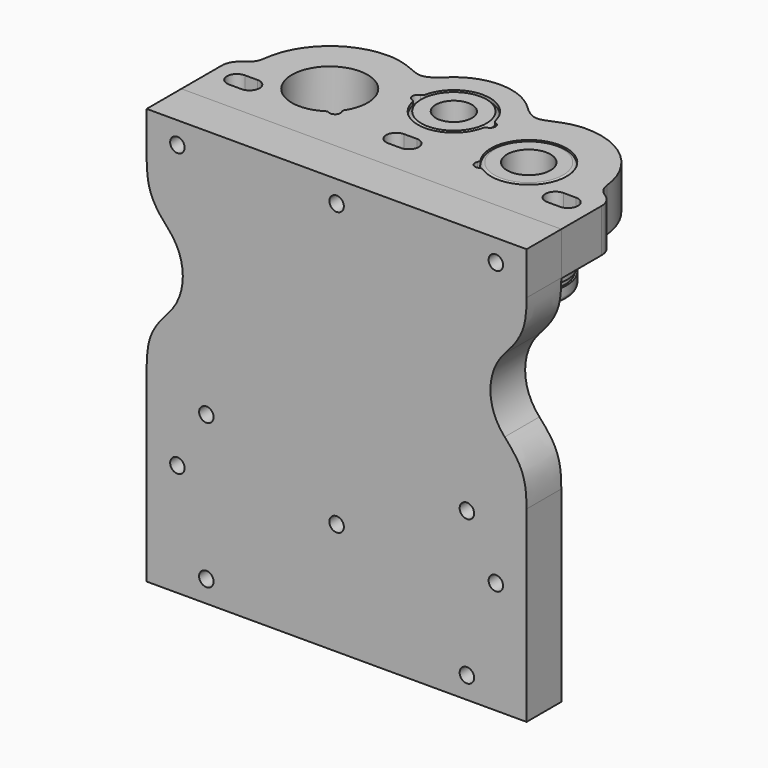
from build123d import *

# Parameters (mm, degrees)
F0_W         = 105
F0_H         = 90
F1_DEPTH     = 12
F3_DEPTH     = 12
F4_R         = 5
F5_R         = 10.5
F5_R_2       = 6
F6_DEPTH     = 30
F8_START     = -3.5
F7_R         = 13.9480454754
F7_R_2       = 10
F8_DEPTH     = 1.3
F10_START    = -3.5
F9_R         = 14.6955703702
F9_R_2       = 10
F10_DEPTH    = 1.3
F11_R        = 1
F12_W        = 105
F12_H        = 25
F13_DEPTH    = 12
F14_R        = 10
F14_R_2      = 5
F15_DEPTH    = 25
F16_R        = 2
F17_DEPTH    = 25
F18_SIZE     = 1
F19_R        = 15
F20_DEPTH    = 25
F21_T1_DEPTH = 69.741647668


# Not quite as in the source:
# - a fillet or chamfer that OpenCascade refuses, or shapes differently, is made with other operations: its cross-section is extruded or revolved along the edge and cut away or added


with BuildPart() as f1:
    # F0 (on Front) → F1 (new body)
    with BuildSketch(Plane.XZ):
        with Locations((0, 45)):
            Rectangle(F0_W, F0_H)
    extrude(amount=-F1_DEPTH)

    # F12 (on face) → F13 (join, through all)
    with BuildSketch(Plane.XZ):
        with Locations((0, -12.5)):
            Rectangle(F12_W, F12_H)
    extrude(amount=-F13_DEPTH)


with BuildPart() as f3:
    # F2 (on face) → F3 (new body)
    with BuildSketch(Plane.XY.offset(90)):
        with BuildLine():
            Line((52.5, 28.5), (47.4999980907, 32))
            ThreePointArc((47.4999980907, 32), (41.6421337144, 46.1421356237), (27.4999980907, 52))
            add(Edge.make_bspline(
                [(11.1242977306, 52), (13.1569224157, 50.0337806808), (16.8978786945, 47.5177026437), (21.9085912172, 52), (27.4999980907, 52)],
                knots=[0, 0, 0, 0, 0.4241441638, 1, 1, 1, 1], degree=3))
            ThreePointArc((11.1242977306, 52), (0, 56.5), (-11.1242977306, 52))
            add(Edge.make_bspline(
                [(-11.1242977306, 52), (-13.1569224157, 50.0337806808), (-16.8978786945, 47.5177026437), (-21.9085912172, 52), (-27.4999980907, 52)],
                knots=[0, 0, 0, 0, 0.4241441638, 1, 1, 1, 1], degree=3))
            ThreePointArc((-27.4999980907, 52), (-41.6421337144, 46.1421356237), (-47.4999980907, 32))
            Line((-47.4999980907, 32), (-52.5, 28.5))
            Line((-52.5, 28.5), (-52.5, 12))
            Line((-52.5, 12), (-47.5, 12))
            Line((-47.5, 12), (47.5, 12))
            Line((47.5, 12), (52.5, 12))
            Line((52.5, 12), (52.5, 28.5))
        make_face()
        with BuildLine():
            Line((-45.75, 25.5), (-42.25, 25.5))
            ThreePointArc((-42.25, 25.5), (-39.5, 22.75), (-42.25, 20))
            Line((-42.25, 20), (-45.75, 20))
            ThreePointArc((-45.75, 20), (-48.5, 22.75), (-45.75, 25.5))
        make_face(mode=Mode.SUBTRACT)
        with BuildLine():
            ThreePointArc((-20.7869945386, 23.2632266648), (-21.2971382344, 23.3755438907), (-21.794316347, 23.2153075842))
            ThreePointArc((-21.794316347, 23.2153075842), (-34.9069416236, 39.4069435329), (-18.7153056748, 26.2943182564))
            ThreePointArc((-18.7153056748, 26.2943182564), (-18.8755419814, 25.7971401438), (-18.7632247555, 25.286996448))
            ThreePointArc((-18.7632247555, 25.286996448), (-19.0323943859, 23.5323962953), (-20.7869945386, 23.2632266648))
        make_face(mode=Mode.SUBTRACT)
        with BuildLine():
            ThreePointArc((-1.75, 20), (-4.5, 22.75), (-1.75, 25.5))
            Line((-1.75, 25.5), (1.75, 25.5))
            ThreePointArc((1.75, 25.5), (4.5, 22.75), (1.75, 20))
            Line((1.75, 20), (-1.75, 20))
        make_face(mode=Mode.SUBTRACT)
        with BuildLine():
            ThreePointArc((42.25, 20), (39.5, 22.75), (42.25, 25.5))
            Line((42.25, 25.5), (45.75, 25.5))
            ThreePointArc((45.75, 25.5), (48.5, 22.75), (45.75, 20))
            Line((45.75, 20), (42.25, 20))
        make_face(mode=Mode.SUBTRACT)
        with BuildLine():
            ThreePointArc((18.7153056748, 26.2943182564), (34.9069416236, 39.4069435329), (21.794316347, 23.2153075842))
            ThreePointArc((21.794316347, 23.2153075842), (21.2971382344, 23.3755438907), (20.7869945386, 23.2632266648))
            ThreePointArc((20.7869945386, 23.2632266648), (19.0323943859, 23.5323962953), (18.7632247555, 25.286996448))
            ThreePointArc((18.7632247555, 25.286996448), (18.8755419814, 25.7971401438), (18.7153056748, 26.2943182564))
        make_face(mode=Mode.SUBTRACT)
        with BuildLine():
            ThreePointArc((9.7358200456, 38.3287254802), (0, 30.525), (-9.7358200456, 38.3287254802))
            ThreePointArc((-9.7358200456, 38.3287254802), (-9.9771083652, 38.7894094573), (-10.4171052632, 39.0666323095))
            ThreePointArc((-10.4171052632, 39.0666323095), (-11.475, 40.5), (-10.4171052632, 41.9333676905))
            ThreePointArc((-10.4171052632, 41.9333676905), (-9.9771083652, 42.2105905427), (-9.7358200456, 42.6712745198))
            ThreePointArc((-9.7358200456, 42.6712745198), (0, 50.475), (9.7358200456, 42.6712745198))
            ThreePointArc((9.7358200456, 42.6712745198), (9.9771083652, 42.2105905427), (10.4171052632, 41.9333676905))
            ThreePointArc((10.4171052632, 41.9333676905), (11.475, 40.5), (10.4171052632, 39.0666323095))
            ThreePointArc((10.4171052632, 39.0666323095), (9.9771083652, 38.7894094573), (9.7358200456, 38.3287254802))
        make_face(mode=Mode.SUBTRACT)
    extrude(amount=-F3_DEPTH)

    # F4
    f4_edges = [f3.edges().sort_by_distance(p)[0] for p in [
        (-47.499998, 32, 84),
        (-52.5, 28.5, 84),
        (47.499998, 32, 84),
        (52.5, 28.5, 84),
    ]]
    fillet(f4_edges, radius=F4_R)


with BuildPart() as f6:
    # F5 (on face) → F6 (new body)
    with BuildSketch(Plane.XY.offset(90)):
        with Locations((27.4999980907, 32)):
            Circle(F5_R)
        with Locations((27.4999980907, 32)):
            Circle(F5_R_2, mode=Mode.SUBTRACT)
    extrude(amount=-F6_DEPTH)

    # F7 (on face) → F8 (cut)
    with BuildSketch(Plane.XY.offset(90).offset(F8_START)):
        with Locations((27.4999980907, 32)):
            Circle(F7_R)
        with Locations((27.4999980907, 32)):
            Circle(F7_R_2, mode=Mode.SUBTRACT)
    extrude(amount=-F8_DEPTH, mode=Mode.SUBTRACT)

    # F9 (on face) → F10 (cut)
    with BuildSketch(Plane(origin=(0, 0, 60), x_dir=(1, 0, 0), z_dir=(0, 0, -1)).offset(F10_START)):
        with Locations((27.4999980907, -32)):
            Circle(F9_R)
        with Locations((27.4999980907, -32)):
            Circle(F9_R_2, mode=Mode.SUBTRACT)
    extrude(amount=-F10_DEPTH, mode=Mode.SUBTRACT)

    # F11
    f11_edges = [f6.edges().sort_by_distance(p)[0] for p in [
        (16.999998, 32, 90),
        (16.999998, 32, 60),
    ]]
    fillet(f11_edges, radius=F11_R)


with BuildPart() as f15:
    # F14 (on face) → F15 (new body)
    with BuildSketch(Plane.XY.offset(90)):
        with Locations((0, 40.5)):
            Circle(F14_R)
        with Locations((0, 40.5)):
            Circle(F14_R_2, mode=Mode.SUBTRACT)
    extrude(amount=-F15_DEPTH)

    # F18
    f18_edges = [f15.edges().sort_by_distance(p)[0] for p in [
        (-10, 40.5, 65),
        (-10, 40.5, 90),
    ]]
    chamfer(f18_edges, length=F18_SIZE)


with BuildPart() as f17_tool:
    # F16 (on face) → F17 (new body)
    with BuildSketch(Plane.XZ):
        with Locations((-44, 84)):
            Circle(F16_R)
        with Locations((44, 84)):
            Circle(F16_R)
        with Locations((0, 84)):
            Circle(F16_R)
        with Locations((44, 6)):
            Circle(F16_R)
        with Locations((0, 6)):
            Circle(F16_R)
        with Locations((-44, 6)):
            Circle(F16_R)
        with Locations((-36, -19)):
            Circle(F16_R)
        with Locations((36, -19)):
            Circle(F16_R)
        with Locations((36, 21)):
            Circle(F16_R)
        with Locations((-36, 21)):
            Circle(F16_R)
    extrude(amount=-F17_DEPTH)


with BuildPart() as f1_1:
    add(f1.part)

    # F17: cut by f17_tool
    add(f17_tool.part, mode=Mode.SUBTRACT)

    # F19 (on face) → F20 (cut)
    with BuildSketch(Plane.XZ):
        with Locations((-57.5, 52.5)):
            Circle(F19_R)
        with Locations((57.5, 52.5)):
            Circle(F19_R)
    extrude(amount=-F20_DEPTH, mode=Mode.SUBTRACT)

    # F21: fillet of radius 23 on 4 edges, made by hand

    # F21_s2 → F21_t1 (cut)
    with BuildSketch(Plane.XZ.offset(-40.870823834)):
        with BuildLine():
            add(Edge.make_bspline(
                [(-52.5, 78.1904651573), (-52.5, 69.2377272995), (-46.4473684211, 62.6409730884)],
                knots=[0, 0, 0, 1, 1, 1], degree=2, weights=[1, 1.5, 1]))
            ThreePointArc((-46.4473684211, 62.6409730884), (-49.2281156584, 65.0130303859), (-52.5, 66.6421356237))
            Line((-52.5, 66.6421356237), (-52.5, 78.1904651573))
        make_face()
        with BuildLine():
            add(Edge.make_bspline(
                [(-52.5, 26.8095348427), (-52.5, 35.7622727005), (-46.4473684211, 42.3590269116)],
                knots=[0, 0, 0, 1, 1, 1], degree=2, weights=[1, 1.5, 1]))
            ThreePointArc((-46.4473684211, 42.3590269116), (-49.2281156584, 39.9869696141), (-52.5, 38.3578643763))
            Line((-52.5, 38.3578643763), (-52.5, 26.8095348427))
        make_face()
        with BuildLine():
            add(Edge.make_bspline(
                [(52.5, 78.1904651573), (52.5, 69.2377272995), (46.4473684211, 62.6409730884)],
                knots=[0, 0, 0, 1, 1, 1], degree=2, weights=[1, 1.5, 1]))
            ThreePointArc((46.4473684211, 62.6409730884), (49.2281156584, 65.0130303859), (52.5, 66.6421356237))
            Line((52.5, 66.6421356237), (52.5, 78.1904651573))
        make_face()
        with BuildLine():
            add(Edge.make_bspline(
                [(46.4473684211, 42.3590269116), (52.5, 35.7622727005), (52.5, 26.8095348427)],
                knots=[0, 0, 0, 1, 1, 1], degree=2, weights=[1, 1.5, 1]))
            Line((52.5, 26.8095348427), (52.5, 38.3578643763))
            ThreePointArc((52.5, 38.3578643763), (49.2281156584, 39.9869696141), (46.4473684211, 42.3590269116))
        make_face()
    extrude(amount=F21_T1_DEPTH, mode=Mode.SUBTRACT)


with BuildPart() as f3_1:
    add(f3.part)

    # F17: cut by f17_tool
    add(f17_tool.part, mode=Mode.SUBTRACT)


solid = Compound([f6.part, f15.part, f1_1.part, f3_1.part])
